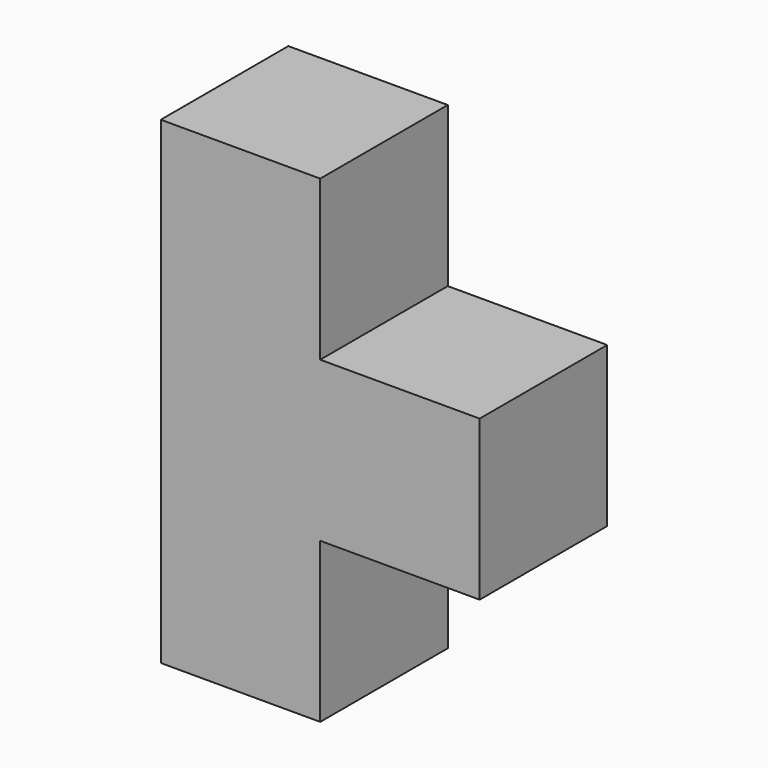
from build123d import *

# Parameters (mm, degrees)
F1_W     = 50.8
F1_H     = 76.2
F2_DEPTH = 25.4
F3_W     = 25.4
F3_H     = 25.4
F4_DEPTH = 25.4
F5_W     = 25.4
F5_H     = 25.4
F6_DEPTH = 25.4


# Not quite as in the source:
# - a variable given as a bare number and used for a length is read in inches; the dataset says mm whatever the document's units were


with BuildPart() as f2:
    # F1 (on Front) → F2 (new body)
    with BuildSketch(Plane.XZ):
        Rectangle(F1_W, F1_H)
    extrude(amount=F2_DEPTH)

    # F3 (on face) → F4 (cut)
    with BuildSketch(Plane.XZ.offset(25.4)):
        with Locations((12.7, 25.4)):
            Rectangle(F3_W, F3_H)
    extrude(amount=-F4_DEPTH, mode=Mode.SUBTRACT)

    # F5 (on face) → F6 (cut)
    with BuildSketch(Plane.XZ.offset(25.4)):
        with Locations((12.7, -25.4)):
            Rectangle(F5_W, F5_H)
    extrude(amount=-F6_DEPTH, mode=Mode.SUBTRACT)


solid = f2.part
